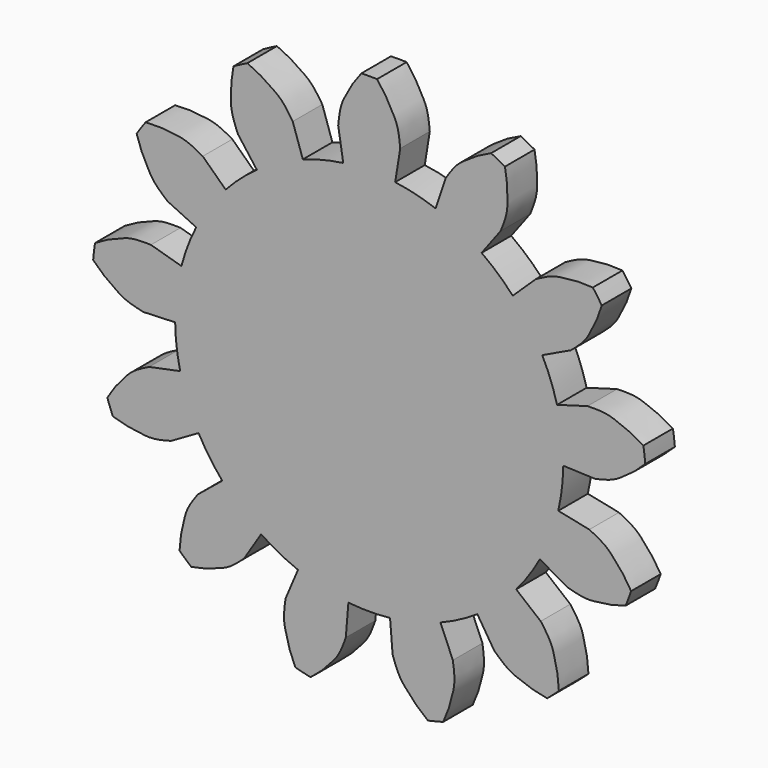
from build123d import *

# Parameters (mm, degrees)
F2_DEPTH        = 20
F2_COPIES_COUNT = 13
F4_DEPTH        = 20


# Not quite as in the source:
# - a pattern or mirror of a feature is missing from the dataset's text; its kind, count and spacing are read off the source's solid


with BuildPart() as f2:
    # F1 (on Front) → F2 (new body)
    with BuildSketch(Plane.XZ):
        with BuildLine():
            ThreePointArc((-14.0470065876, 104.0561464111), (0, 105), (14.0470065876, 104.0561464111))
            Line((14.0470065876, 104.0561464111), (16.7773367506, 121.0024649167))
            add(Edge.make_bspline(
                [(4.2468093523, 149.9398699824), (4.4290412164, 149.7210246606), (8.7826343305, 144.3294696938), (13.1358942294, 135.9586969958), (15.9340407786, 130.266903883), (16.7579313288, 121.3103558316), (16.7773367506, 121.0024649167)],
                knots=[0, 0, 0, 0, 0.2214991664, 0.5040555337, 0.7473622312, 1, 1, 1, 1], degree=3))
            ThreePointArc((4.2468093523, 149.9398699824), (0, 150), (-4.2468093523, 149.9398699824))
            add(Edge.make_bspline(
                [(-4.2468093523, 149.9398699824), (-4.4290412164, 149.7210246606), (-8.7826343305, 144.3294696938), (-13.1358942294, 135.9586969958), (-15.9340407786, 130.266903883), (-16.7579313288, 121.3103558316), (-16.7773367506, 121.0024649167)],
                knots=[0, 0, 0, 0, 0.2214991664, 0.5040555337, 0.7473622312, 1, 1, 1, 1], degree=3))
            Line((-16.7773367506, 121.0024649167), (-14.0470065876, 104.0561464111))
        make_face()
    extrude(amount=F2_DEPTH)


with BuildPart() as f2_copies_1:
    # F2_copies: instance of F2
    add(f2.part.rotate(Axis((0, 0, 0), (0, 1, 0)), 1 * 360 / F2_COPIES_COUNT))


with BuildPart() as f2_copies_2:
    # F2_copies: instance of F2
    add(f2.part.rotate(Axis((0, 0, 0), (0, 1, 0)), 2 * 360 / F2_COPIES_COUNT))


with BuildPart() as f2_copies_3:
    # F2_copies: instance of F2
    add(f2.part.rotate(Axis((0, 0, 0), (0, 1, 0)), 3 * 360 / F2_COPIES_COUNT))


with BuildPart() as f2_copies_4:
    # F2_copies: instance of F2
    add(f2.part.rotate(Axis((0, 0, 0), (0, 1, 0)), 4 * 360 / F2_COPIES_COUNT))


with BuildPart() as f2_copies_5:
    # F2_copies: instance of F2
    add(f2.part.rotate(Axis((0, 0, 0), (0, 1, 0)), 5 * 360 / F2_COPIES_COUNT))


with BuildPart() as f2_copies_6:
    # F2_copies: instance of F2
    add(f2.part.rotate(Axis((0, 0, 0), (0, 1, 0)), 6 * 360 / F2_COPIES_COUNT))


with BuildPart() as f2_copies_7:
    # F2_copies: instance of F2
    add(f2.part.rotate(Axis((0, 0, 0), (0, 1, 0)), 7 * 360 / F2_COPIES_COUNT))


with BuildPart() as f2_copies_8:
    # F2_copies: instance of F2
    add(f2.part.rotate(Axis((0, 0, 0), (0, 1, 0)), 8 * 360 / F2_COPIES_COUNT))


with BuildPart() as f2_copies_9:
    # F2_copies: instance of F2
    add(f2.part.rotate(Axis((0, 0, 0), (0, 1, 0)), 9 * 360 / F2_COPIES_COUNT))


with BuildPart() as f2_copies_10:
    # F2_copies: instance of F2
    add(f2.part.rotate(Axis((0, 0, 0), (0, 1, 0)), 10 * 360 / F2_COPIES_COUNT))


with BuildPart() as f2_copies_11:
    # F2_copies: instance of F2
    add(f2.part.rotate(Axis((0, 0, 0), (0, 1, 0)), 11 * 360 / F2_COPIES_COUNT))


with BuildPart() as f2_copies_12:
    # F2_copies: instance of F2
    add(f2.part.rotate(Axis((0, 0, 0), (0, 1, 0)), 12 * 360 / F2_COPIES_COUNT))


with BuildPart() as f2_1:
    add(f2.part)

    add(f2_copies_1.part)  # F4 merges F2_copies_1

    add(f2_copies_2.part)  # F4 merges F2_copies_2

    add(f2_copies_3.part)  # F4 merges F2_copies_3

    add(f2_copies_4.part)  # F4 merges F2_copies_4

    add(f2_copies_5.part)  # F4 merges F2_copies_5

    add(f2_copies_6.part)  # F4 merges F2_copies_6

    add(f2_copies_7.part)  # F4 merges F2_copies_7

    add(f2_copies_8.part)  # F4 merges F2_copies_8

    add(f2_copies_9.part)  # F4 merges F2_copies_9

    add(f2_copies_10.part)  # F4 merges F2_copies_10

    add(f2_copies_11.part)  # F4 merges F2_copies_11

    add(f2_copies_12.part)  # F4 merges F2_copies_12
    # F1 (on Front) → F4 (join)
    with BuildSketch(Plane.XZ):
        with BuildLine():
            ThreePointArc((-14.0470065876, 104.0561464111), (-69.1016074643, -79.0567381432), (105, 0))
            ThreePointArc((105, 0), (79.0567381432, 69.1016074643), (14.0470065876, 104.0561464111))
            ThreePointArc((14.0470065876, 104.0561464111), (0, 105), (-14.0470065876, 104.0561464111))
        make_face()
    extrude(amount=F4_DEPTH)


solid = f2_1.part
